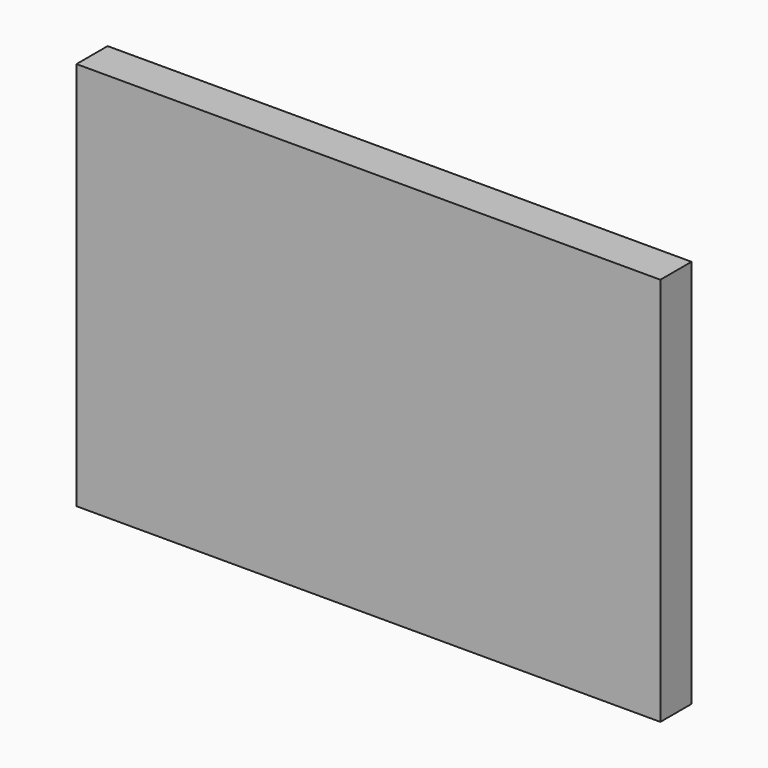
from build123d import *

# Parameters (mm, degrees)
F0_W     = 45
F0_H     = 30
F1_DEPTH = 1.5
F2_D     = 5
F2_DEPTH = 1.501


with BuildPart() as f1:
    # F0 (on Front) → F1 (new body, symmetric)
    with BuildSketch(Plane.XZ):
        with Locations((-9.7826488498, 10.1560708135)):
            Rectangle(F0_W, F0_H)
    extrude(amount=F1_DEPTH, both=True)

    # F2 (through all, one way)
    with BuildSketch(Plane.XZ):
        with Locations((-27.2826488498, 10.1560708135)):
            Circle(F2_D / 2)
    extrude(amount=-F2_DEPTH, mode=Mode.SUBTRACT)


solid = f1.part
